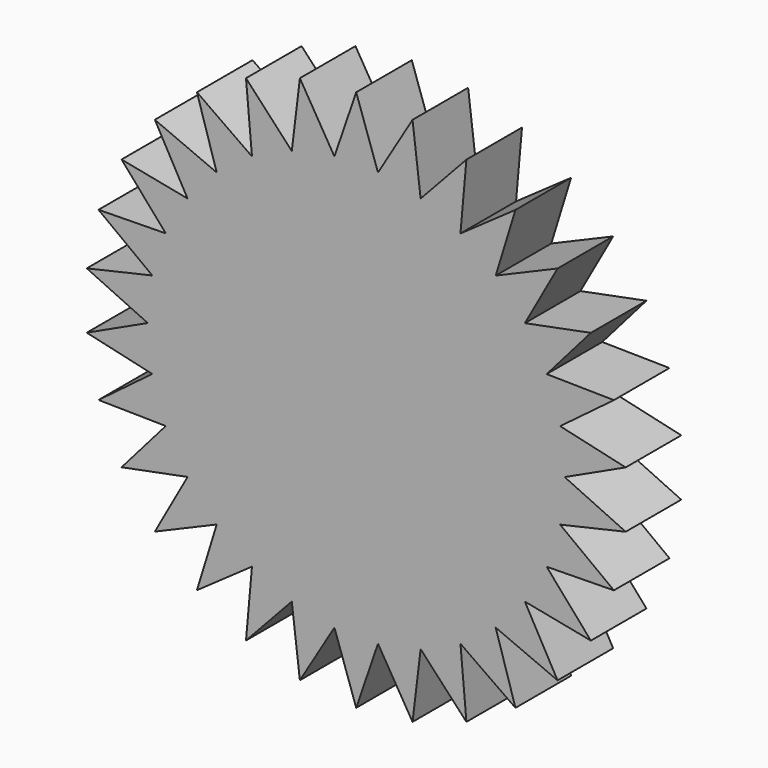
from build123d import *

# Parameters (mm, degrees)
F0_R            = 60
F1_DEPTH        = 20
F3_DEPTH        = 20
F3_COPIES_COUNT = 30


# Not quite as in the source:
# - a pattern or mirror of a feature is missing from the dataset's text; its kind, count and spacing are read off the source's solid


with BuildPart() as f1:
    # F0 (on Front) → F1 (new body)
    with BuildSketch(Plane.XZ):
        Circle(F0_R)
    extrude(amount=F1_DEPTH)

    # F2 (on face) → F3 (join)
    with BuildSketch(Plane.XZ.offset(20)):
        Polygon((0, 77.9763460159), (-6.2717077961, 59.6713137221), (6.2717077961, 59.6713137221), align=None)
    f3 = extrude(amount=-F3_DEPTH)

    # F3_copies: F3 ×30 about axis
    f3_copies_axis = Axis((0, 0, 0), (0, 1, 0))
    for i in range(1, F3_COPIES_COUNT):
        add(f3.rotate(f3_copies_axis, i * 360 / F3_COPIES_COUNT))


solid = f1.part
